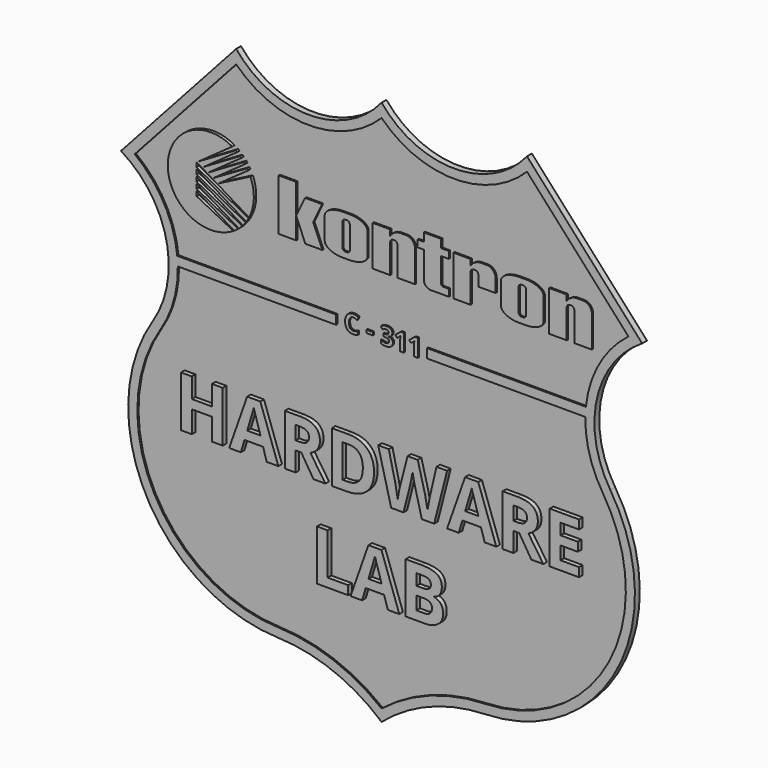
from build123d import *

# Parameters (mm, degrees)
F1_DEPTH      = 1.5
F2_DEPTH      = 0.5
F4_DEPTH      = 0.5
F5_TEXT_SIZE  = 8.0693968126
F6_DEPTH      = 0.5
F7_TEXT_SIZE  = 23.5255677177
F8_DEPTH      = 1.5
F9_DEPTH      = 1
F10_TEXT_SIZE = 23.3264580951
F11_DEPTH     = 1.5


# Not quite as in the source:
# - Text() gives the source's letters only with a copy of the font that has no kerning and outlines rounded to 1/6400 em; it was checked with that copy


with BuildPart() as f1:
    # F0 (on Front) → F1 (new body)
    with BuildSketch(Plane.XZ):
        with BuildLine():
            Line((156.4623748512, 13), (118.4623748512, 55))
            ThreePointArc((118.4623748512, 55), (94.4623748512, 43.6214168703), (70.4623748512, 55))
            ThreePointArc((70.4623748512, 55), (46.4623748512, 43.6214168703), (22.4623748512, 55))
            Line((22.4623748512, 55), (-15.5376251488, 13))
            ThreePointArc((-15.5376251488, 13), (-0.6111192408, -7.7912323471), (-5.0376251488, -33))
            ThreePointArc((-5.0376251488, -33), (-7.3094849926, -84.3223540765), (36.2328714478, -111.5842060078))
            ThreePointArc((36.2328714478, -111.5842060078), (54.4964482859, -115.3218559064), (70.4623748512, -124.9456521739))
            ThreePointArc((70.4623748512, -124.9456521739), (86.4283014165, -115.3218559064), (104.6918782546, -111.5842060078))
            ThreePointArc((104.6918782546, -111.5842060078), (148.234234695, -84.3223540765), (145.9623748512, -33))
            ThreePointArc((145.9623748512, -33), (141.5358689433, -7.7912323471), (156.4623748512, 13))
        make_face()
        with BuildLine():
            ThreePointArc((27.5723614134, 19.745571844), (28.6903368347, 13.6762247438), (27.1279654253, 7.7058111194))
            Line((27.1279654253, 7.7058111194), (9.8, 18.2))
            Line((9.8, 18.2), (9.8, 16.7))
            Line((9.8, 16.7), (26.9879537237, 7.4404873108))
            ThreePointArc((26.9879537237, 7.4404873108), (26.614342533, 6.7917137614), (26.2070574809, 6.1635327949))
            Line((26.2070574809, 6.1635327949), (9.8, 16.1))
            Line((9.8, 16.1), (9.8, 14.6))
            Line((9.8, 14.6), (26.0346697714, 5.9180078927))
            ThreePointArc((26.0346697714, 5.9180078927), (25.5780217671, 5.3164515126), (25.0900363512, 4.7400248372))
            Line((25.0900363512, 4.7400248372), (9.8, 14))
            Line((9.8, 14), (9.8, 12.5))
            Line((9.8, 12.5), (24.8878254934, 4.5184153406))
            ThreePointArc((24.8878254934, 4.5184153406), (24.3423672704, 3.9643853866), (23.7674037222, 3.4410396297))
            Line((23.7674037222, 3.4410396297), (9.8, 11.9))
            Line((9.8, 11.9), (9.8, 10.4))
            Line((9.8, 10.4), (23.5380462181, 3.2476614114))
            ThreePointArc((23.5380462181, 3.2476614114), (22.8915080931, 2.7447570116), (22.2170485866, 2.2799680742))
            Line((22.2170485866, 2.2799680742), (9.8, 9.8))
            Line((9.8, 9.8), (9.8, 8.3))
            Line((9.8, 8.3), (21.9635087632, 2.1196011265))
            ThreePointArc((21.9635087632, 2.1196011265), (0.3018885432, 13.968416191), (21.5655593046, 26.5173808788))
            Line((21.5655593046, 26.5173808788), (10.3, 18.4817355208))
            Line((10.3, 18.4817355208), (22.7054346966, 25.7892554308))
            ThreePointArc((22.7054346966, 25.7892554308), (22.9484467099, 25.6133145137), (23.1876874226, 25.4322788092))
            Line((23.1876874226, 25.4322788092), (12, 17.4521789249))
            Line((12, 17.4521789249), (24.1596372379, 24.6082375277))
            ThreePointArc((24.1596372379, 24.6082375277), (24.3773735981, 24.4018376189), (24.5907007992, 24.1908837137))
            Line((24.5907007992, 24.1908837137), (13.7, 16.422622329))
            Line((13.7, 16.422622329), (25.420447696, 23.2765534273))
            ThreePointArc((25.420447696, 23.2765534273), (25.6097684786, 23.043813903), (25.7941299736, 22.8071265901))
            Line((25.7941299736, 22.8071265901), (15.4, 15.3930657331))
            Line((15.4, 15.3930657331), (26.4951006995, 21.79983942))
            ThreePointArc((26.4951006995, 21.79983942), (26.6529834417, 21.5447255541), (26.8054412158, 21.2863330774))
            Line((26.8054412158, 21.2863330774), (17.1, 14.3635091373))
            Line((17.1, 14.3635091373), (27.5723614134, 19.745571844))
        make_face(mode=Mode.SUBTRACT)
        Polygon((42.3, 5.8), (36.5, 5.8), (36.5, 22.8), (42.3, 22.8), (42.3, 13.1), (45.2263955314, 19.1), (50.8263955314, 19.1), (47.9, 12.9), (50.9137711951, 5.8), (45.3137711951, 5.8), (42.3, 12.9), align=None, mode=Mode.SUBTRACT)
        with BuildLine():
            Line((51.7, 8.8), (51.7, 16.1))
            add(Edge.make_bspline(
                [(57.5, 19.1), (51.7, 19.1), (51.7, 16.1)],
                knots=[4.7123889804, 4.7123889804, 4.7123889804, 6.2831853072, 6.2831853072, 6.2831853072], degree=2, weights=[1, 0.7071067812, 1]))
            Line((57.5, 19.1), (60, 19.1))
            add(Edge.make_bspline(
                [(65.8, 16.1), (65.8, 19.1), (60, 19.1)],
                knots=[3.1415926536, 3.1415926536, 3.1415926536, 4.7123889804, 4.7123889804, 4.7123889804], degree=2, weights=[1, 0.7071067812, 1]))
            Line((65.8, 16.1), (65.8, 8.8))
            add(Edge.make_bspline(
                [(60, 5.8), (65.8, 5.8), (65.8, 8.8)],
                knots=[4.7123889804, 4.7123889804, 4.7123889804, 6.2831853072, 6.2831853072, 6.2831853072], degree=2, weights=[1, 0.7071067812, 1]))
            Line((60, 5.8), (57.5, 5.8))
            add(Edge.make_bspline(
                [(51.7, 8.8), (51.7, 5.8), (57.5, 5.8)],
                knots=[3.1415926536, 3.1415926536, 3.1415926536, 4.7123889804, 4.7123889804, 4.7123889804], degree=2, weights=[1, 0.7071067812, 1]))
        make_face(mode=Mode.SUBTRACT)
        with BuildLine():
            Line((67.5, 5.8), (67.5, 19.1))
            Line((67.5, 19.1), (73.3, 19.1))
            Line((73.3, 19.1), (73.3, 17.2))
            ThreePointArc((73.3, 17.2), (74.7550500371, 18.5928498393), (76.7044089061, 19.1))
            Line((76.7044089061, 19.1), (78.6002400503, 19.1))
            ThreePointArc((78.6002400503, 19.1), (80.6508497158, 18.2506096654), (81.5002400503, 16.2))
            Line((81.5002400503, 16.2), (81.5002400503, 5.8))
            Line((81.5002400503, 5.8), (75.7002400503, 5.8))
            Line((75.7002400503, 5.8), (75.7002400503, 15.4))
            ThreePointArc((75.7002400503, 15.4), (75.4073468315, 16.1071067812), (74.7002400503, 16.4))
            Line((74.7002400503, 16.4), (74.3, 16.4))
            ThreePointArc((74.3, 16.4), (73.5928932188, 16.1071067812), (73.3, 15.4))
            Line((73.3, 15.4), (73.3, 5.8))
            Line((73.3, 5.8), (67.5, 5.8))
        make_face(mode=Mode.SUBTRACT)
        with BuildLine():
            Line((84.4002400503, 16.8), (82.4002400503, 16.8))
            Line((82.4002400503, 16.8), (82.4002400503, 19.1))
            Line((82.4002400503, 19.1), (84.4002400503, 19.1))
            Line((84.4002400503, 19.1), (84.4002400503, 21.8))
            Line((84.4002400503, 21.8), (90.1002400503, 21.8))
            Line((90.1002400503, 21.8), (90.1002400503, 19.1))
            Line((90.1002400503, 19.1), (92.6768170513, 19.1))
            Line((92.6768170513, 19.1), (92.6768170513, 16.8))
            Line((92.6768170513, 16.8), (90.1002400503, 16.8))
            Line((90.1002400503, 16.8), (90.1002400503, 8.8))
            ThreePointArc((90.1002400503, 8.8), (90.3052653035, 8.3050252532), (90.8002400503, 8.1))
            Line((90.8002400503, 8.1), (92.6768170513, 8.1))
            Line((92.6768170513, 8.1), (92.6768170513, 5.8))
            Line((92.6768170513, 5.8), (86.7002400503, 5.8))
            ThreePointArc((86.7002400503, 5.8), (85.0738944536, 6.4736544033), (84.4002400503, 8.1))
            Line((84.4002400503, 8.1), (84.4002400503, 16.8))
        make_face(mode=Mode.SUBTRACT)
        with BuildLine():
            Line((94.1768170513, 5.8), (94.1768170513, 19.1))
            Line((94.1768170513, 19.1), (99.8768170513, 19.1))
            Line((99.8768170513, 19.1), (99.8768170513, 17.2))
            ThreePointArc((99.8768170513, 17.2), (101.3318670884, 18.5928498393), (103.2812259574, 19.1))
            Line((103.2812259574, 19.1), (105.1768170513, 19.1))
            ThreePointArc((105.1768170513, 19.1), (107.2274267167, 18.2506096654), (108.0768170513, 16.2))
            Line((108.0768170513, 16.2), (108.0768170513, 11.9))
            Line((108.0768170513, 11.9), (102.3768170513, 11.9))
            Line((102.3768170513, 11.9), (102.3768170513, 15.4))
            ThreePointArc((102.3768170513, 15.4), (102.0839238324, 16.1071067812), (101.3768170513, 16.4))
            Line((101.3768170513, 16.4), (100.8768170513, 16.4))
            ThreePointArc((100.8768170513, 16.4), (100.1697102701, 16.1071067812), (99.8768170513, 15.4))
            Line((99.8768170513, 15.4), (99.8768170513, 5.8))
            Line((99.8768170513, 5.8), (94.1768170513, 5.8))
        make_face(mode=Mode.SUBTRACT)
        with BuildLine():
            add(Edge.make_bspline(
                [(123.9768170513, 16.1), (123.9768170513, 19.1), (118.1768170513, 19.1)],
                knots=[0, 0, 0, 1.5707963268, 1.5707963268, 1.5707963268], degree=2, weights=[1, 0.7071067812, 1]))
            Line((123.9768170513, 16.1), (123.9768170513, 8.8))
            add(Edge.make_bspline(
                [(118.1768170513, 5.8), (123.9768170513, 5.8), (123.9768170513, 8.8)],
                knots=[4.7123889804, 4.7123889804, 4.7123889804, 6.2831853072, 6.2831853072, 6.2831853072], degree=2, weights=[1, 0.7071067812, 1]))
            Line((118.1768170513, 5.8), (115.6768170513, 5.8))
            add(Edge.make_bspline(
                [(109.8768170513, 8.8), (109.8768170513, 5.8), (115.6768170513, 5.8)],
                knots=[3.1415926536, 3.1415926536, 3.1415926536, 4.7123889804, 4.7123889804, 4.7123889804], degree=2, weights=[1, 0.7071067812, 1]))
            Line((109.8768170513, 8.8), (109.8768170513, 16.1))
            add(Edge.make_bspline(
                [(115.6768170513, 19.1), (109.8768170513, 19.1), (109.8768170513, 16.1)],
                knots=[4.7123889804, 4.7123889804, 4.7123889804, 6.2831853072, 6.2831853072, 6.2831853072], degree=2, weights=[1, 0.7071067812, 1]))
            Line((115.6768170513, 19.1), (118.1768170513, 19.1))
        make_face(mode=Mode.SUBTRACT)
        with BuildLine():
            Line((125.7768170513, 5.8), (125.7768170513, 19.1))
            Line((125.7768170513, 19.1), (131.5768170513, 19.1))
            Line((131.5768170513, 19.1), (131.5768170513, 17.2))
            ThreePointArc((131.5768170513, 17.2), (133.0318670884, 18.5928498393), (134.9812259574, 19.1))
            Line((134.9812259574, 19.1), (136.9768170513, 19.1))
            ThreePointArc((136.9768170513, 19.1), (139.0274267167, 18.2506096654), (139.8768170513, 16.2))
            Line((139.8768170513, 16.2), (139.8768170513, 5.8))
            Line((139.8768170513, 5.8), (134.0768170513, 5.8))
            Line((134.0768170513, 5.8), (134.0768170513, 15.4))
            ThreePointArc((134.0768170513, 15.4), (133.7839238324, 16.1071067812), (133.0768170513, 16.4))
            Line((133.0768170513, 16.4), (132.5768170513, 16.4))
            ThreePointArc((132.5768170513, 16.4), (131.8697102701, 16.1071067812), (131.5768170513, 15.4))
            Line((131.5768170513, 15.4), (131.5768170513, 5.8))
            Line((131.5768170513, 5.8), (125.7768170513, 5.8))
        make_face(mode=Mode.SUBTRACT)
        with BuildLine():
            Line((9.8, 18.2), (27.1279654253, 7.7058111194))
            ThreePointArc((27.1279654253, 7.7058111194), (28.6903368347, 13.6762247438), (27.5723614134, 19.745571844))
            Line((27.5723614134, 19.745571844), (17.1, 14.3635091373))
            Line((17.1, 14.3635091373), (26.8054412158, 21.2863330774))
            ThreePointArc((26.8054412158, 21.2863330774), (26.6529834417, 21.5447255541), (26.4951006995, 21.79983942))
            Line((26.4951006995, 21.79983942), (15.4, 15.3930657331))
            Line((15.4, 15.3930657331), (25.7941299736, 22.8071265901))
            ThreePointArc((25.7941299736, 22.8071265901), (25.6097684786, 23.043813903), (25.420447696, 23.2765534273))
            Line((25.420447696, 23.2765534273), (13.7, 16.422622329))
            Line((13.7, 16.422622329), (24.5907007992, 24.1908837137))
            ThreePointArc((24.5907007992, 24.1908837137), (24.3773735981, 24.4018376189), (24.1596372379, 24.6082375277))
            Line((24.1596372379, 24.6082375277), (12, 17.4521789249))
            Line((12, 17.4521789249), (23.1876874226, 25.4322788092))
            ThreePointArc((23.1876874226, 25.4322788092), (22.9484467099, 25.6133145137), (22.7054346966, 25.7892554308))
            Line((22.7054346966, 25.7892554308), (10.3, 18.4817355208))
            Line((10.3, 18.4817355208), (21.5655593046, 26.5173808788))
            ThreePointArc((21.5655593046, 26.5173808788), (0.3018885432, 13.968416191), (21.9635087632, 2.1196011265))
            Line((21.9635087632, 2.1196011265), (9.8, 8.3))
            Line((9.8, 8.3), (9.8, 9.8))
            Line((9.8, 9.8), (22.2170485866, 2.2799680742))
            ThreePointArc((22.2170485866, 2.2799680742), (22.8915080931, 2.7447570116), (23.5380462181, 3.2476614114))
            Line((23.5380462181, 3.2476614114), (9.8, 10.4))
            Line((9.8, 10.4), (9.8, 11.9))
            Line((9.8, 11.9), (23.7674037222, 3.4410396297))
            ThreePointArc((23.7674037222, 3.4410396297), (24.3423672704, 3.9643853866), (24.8878254934, 4.5184153406))
            Line((24.8878254934, 4.5184153406), (9.8, 12.5))
            Line((9.8, 12.5), (9.8, 14))
            Line((9.8, 14), (25.0900363512, 4.7400248372))
            ThreePointArc((25.0900363512, 4.7400248372), (25.5780217671, 5.3164515126), (26.0346697714, 5.9180078927))
            Line((26.0346697714, 5.9180078927), (9.8, 14.6))
            Line((9.8, 14.6), (9.8, 16.1))
            Line((9.8, 16.1), (26.2070574809, 6.1635327949))
            ThreePointArc((26.2070574809, 6.1635327949), (26.614342533, 6.7917137614), (26.9879537237, 7.4404873108))
            Line((26.9879537237, 7.4404873108), (9.8, 16.7))
            Line((9.8, 16.7), (9.8, 18.2))
        make_face()
        Polygon((36.5, 22.8), (36.5, 5.8), (42.3, 5.8), (42.3, 12.9), (45.3137711951, 5.8), (50.9137711951, 5.8), (47.9, 12.9), (50.8263955314, 19.1), (45.2263955314, 19.1), (42.3, 13.1), (42.3, 22.8), align=None)
        with BuildLine():
            add(Edge.make_bspline(
                [(57.5, 19.1), (51.7, 19.1), (51.7, 16.1)],
                knots=[4.7123889804, 4.7123889804, 4.7123889804, 6.2831853072, 6.2831853072, 6.2831853072], degree=2, weights=[1, 0.7071067812, 1]))
            Line((51.7, 16.1), (51.7, 8.8))
            add(Edge.make_bspline(
                [(51.7, 8.8), (51.7, 5.8), (57.5, 5.8)],
                knots=[3.1415926536, 3.1415926536, 3.1415926536, 4.7123889804, 4.7123889804, 4.7123889804], degree=2, weights=[1, 0.7071067812, 1]))
            Line((57.5, 5.8), (60, 5.8))
            add(Edge.make_bspline(
                [(60, 5.8), (65.8, 5.8), (65.8, 8.8)],
                knots=[4.7123889804, 4.7123889804, 4.7123889804, 6.2831853072, 6.2831853072, 6.2831853072], degree=2, weights=[1, 0.7071067812, 1]))
            Line((65.8, 8.8), (65.8, 16.1))
            add(Edge.make_bspline(
                [(65.8, 16.1), (65.8, 19.1), (60, 19.1)],
                knots=[3.1415926536, 3.1415926536, 3.1415926536, 4.7123889804, 4.7123889804, 4.7123889804], degree=2, weights=[1, 0.7071067812, 1]))
            Line((60, 19.1), (57.5, 19.1))
        make_face()
        with BuildLine():
            ThreePointArc((58.5, 7.8), (57.7928932188, 8.0928932188), (57.5, 8.8))
            Line((57.5, 8.8), (57.5, 16.1))
            ThreePointArc((57.5, 16.1), (57.7928932188, 16.8071067812), (58.5, 17.1))
            Line((58.5, 17.1), (59, 17.1))
            ThreePointArc((59, 17.1), (59.7071067812, 16.8071067812), (60, 16.1))
            Line((60, 16.1), (60, 8.8))
            ThreePointArc((60, 8.8), (59.7071067812, 8.0928932188), (59, 7.8))
            Line((59, 7.8), (58.5, 7.8))
        make_face(mode=Mode.SUBTRACT)
        with BuildLine():
            Line((73.3, 19.1), (67.5, 19.1))
            Line((67.5, 19.1), (67.5, 5.8))
            Line((67.5, 5.8), (73.3, 5.8))
            Line((73.3, 5.8), (73.3, 15.4))
            ThreePointArc((73.3, 15.4), (73.5928932188, 16.1071067812), (74.3, 16.4))
            Line((74.3, 16.4), (74.7002400503, 16.4))
            ThreePointArc((74.7002400503, 16.4), (75.4073468315, 16.1071067812), (75.7002400503, 15.4))
            Line((75.7002400503, 15.4), (75.7002400503, 5.8))
            Line((75.7002400503, 5.8), (81.5002400503, 5.8))
            Line((81.5002400503, 5.8), (81.5002400503, 16.2))
            ThreePointArc((81.5002400503, 16.2), (80.6508497158, 18.2506096654), (78.6002400503, 19.1))
            Line((78.6002400503, 19.1), (76.7044089061, 19.1))
            ThreePointArc((76.7044089061, 19.1), (74.7550500371, 18.5928498393), (73.3, 17.2))
            Line((73.3, 17.2), (73.3, 19.1))
        make_face()
        with BuildLine():
            Line((82.4002400503, 19.1), (82.4002400503, 16.8))
            Line((82.4002400503, 16.8), (84.4002400503, 16.8))
            Line((84.4002400503, 16.8), (84.4002400503, 8.1))
            ThreePointArc((84.4002400503, 8.1), (85.0738944536, 6.4736544033), (86.7002400503, 5.8))
            Line((86.7002400503, 5.8), (92.6768170513, 5.8))
            Line((92.6768170513, 5.8), (92.6768170513, 8.1))
            Line((92.6768170513, 8.1), (90.8002400503, 8.1))
            ThreePointArc((90.8002400503, 8.1), (90.3052653035, 8.3050252532), (90.1002400503, 8.8))
            Line((90.1002400503, 8.8), (90.1002400503, 16.8))
            Line((90.1002400503, 16.8), (92.6768170513, 16.8))
            Line((92.6768170513, 16.8), (92.6768170513, 19.1))
            Line((92.6768170513, 19.1), (90.1002400503, 19.1))
            Line((90.1002400503, 19.1), (90.1002400503, 21.8))
            Line((90.1002400503, 21.8), (84.4002400503, 21.8))
            Line((84.4002400503, 21.8), (84.4002400503, 19.1))
            Line((84.4002400503, 19.1), (82.4002400503, 19.1))
        make_face()
        with BuildLine():
            Line((57.5, 16.1), (57.5, 8.8))
            ThreePointArc((57.5, 8.8), (57.7928932188, 8.0928932188), (58.5, 7.8))
            Line((58.5, 7.8), (59, 7.8))
            ThreePointArc((59, 7.8), (59.7071067812, 8.0928932188), (60, 8.8))
            Line((60, 8.8), (60, 16.1))
            ThreePointArc((60, 16.1), (59.7071067812, 16.8071067812), (59, 17.1))
            Line((59, 17.1), (58.5, 17.1))
            ThreePointArc((58.5, 17.1), (57.7928932188, 16.8071067812), (57.5, 16.1))
        make_face()
        with BuildLine():
            Line((99.8768170513, 19.1), (94.1768170513, 19.1))
            Line((94.1768170513, 19.1), (94.1768170513, 5.8))
            Line((94.1768170513, 5.8), (99.8768170513, 5.8))
            Line((99.8768170513, 5.8), (99.8768170513, 15.4))
            ThreePointArc((99.8768170513, 15.4), (100.1697102701, 16.1071067812), (100.8768170513, 16.4))
            Line((100.8768170513, 16.4), (101.3768170513, 16.4))
            ThreePointArc((101.3768170513, 16.4), (102.0839238324, 16.1071067812), (102.3768170513, 15.4))
            Line((102.3768170513, 15.4), (102.3768170513, 11.9))
            Line((102.3768170513, 11.9), (108.0768170513, 11.9))
            Line((108.0768170513, 11.9), (108.0768170513, 16.2))
            ThreePointArc((108.0768170513, 16.2), (107.2274267167, 18.2506096654), (105.1768170513, 19.1))
            Line((105.1768170513, 19.1), (103.2812259574, 19.1))
            ThreePointArc((103.2812259574, 19.1), (101.3318670884, 18.5928498393), (99.8768170513, 17.2))
            Line((99.8768170513, 17.2), (99.8768170513, 19.1))
        make_face()
        with BuildLine():
            Line((123.9768170513, 8.8), (123.9768170513, 16.1))
            add(Edge.make_bspline(
                [(123.9768170513, 16.1), (123.9768170513, 19.1), (118.1768170513, 19.1)],
                knots=[0, 0, 0, 1.5707963268, 1.5707963268, 1.5707963268], degree=2, weights=[1, 0.7071067812, 1]))
            Line((118.1768170513, 19.1), (115.6768170513, 19.1))
            add(Edge.make_bspline(
                [(115.6768170513, 19.1), (109.8768170513, 19.1), (109.8768170513, 16.1)],
                knots=[4.7123889804, 4.7123889804, 4.7123889804, 6.2831853072, 6.2831853072, 6.2831853072], degree=2, weights=[1, 0.7071067812, 1]))
            Line((109.8768170513, 16.1), (109.8768170513, 8.8))
            add(Edge.make_bspline(
                [(109.8768170513, 8.8), (109.8768170513, 5.8), (115.6768170513, 5.8)],
                knots=[3.1415926536, 3.1415926536, 3.1415926536, 4.7123889804, 4.7123889804, 4.7123889804], degree=2, weights=[1, 0.7071067812, 1]))
            Line((115.6768170513, 5.8), (118.1768170513, 5.8))
            add(Edge.make_bspline(
                [(118.1768170513, 5.8), (123.9768170513, 5.8), (123.9768170513, 8.8)],
                knots=[4.7123889804, 4.7123889804, 4.7123889804, 6.2831853072, 6.2831853072, 6.2831853072], degree=2, weights=[1, 0.7071067812, 1]))
        make_face()
        with BuildLine():
            Line((115.6768170513, 8.8), (115.6768170513, 16.1))
            ThreePointArc((115.6768170513, 16.1), (115.9697102701, 16.8071067812), (116.6768170513, 17.1))
            Line((116.6768170513, 17.1), (117.1768170513, 17.1))
            ThreePointArc((117.1768170513, 17.1), (117.8839238324, 16.8071067812), (118.1768170513, 16.1))
            Line((118.1768170513, 16.1), (118.1768170513, 8.8))
            ThreePointArc((118.1768170513, 8.8), (117.8839238324, 8.0928932188), (117.1768170513, 7.8))
            Line((117.1768170513, 7.8), (116.6768170513, 7.8))
            ThreePointArc((116.6768170513, 7.8), (115.9697102701, 8.0928932188), (115.6768170513, 8.8))
        make_face(mode=Mode.SUBTRACT)
        with BuildLine():
            ThreePointArc((116.6768170513, 17.1), (115.9697102701, 16.8071067812), (115.6768170513, 16.1))
            Line((115.6768170513, 16.1), (115.6768170513, 8.8))
            ThreePointArc((115.6768170513, 8.8), (115.9697102701, 8.0928932188), (116.6768170513, 7.8))
            Line((116.6768170513, 7.8), (117.1768170513, 7.8))
            ThreePointArc((117.1768170513, 7.8), (117.8839238324, 8.0928932188), (118.1768170513, 8.8))
            Line((118.1768170513, 8.8), (118.1768170513, 16.1))
            ThreePointArc((118.1768170513, 16.1), (117.8839238324, 16.8071067812), (117.1768170513, 17.1))
            Line((117.1768170513, 17.1), (116.6768170513, 17.1))
        make_face()
        with BuildLine():
            Line((131.5768170513, 19.1), (125.7768170513, 19.1))
            Line((125.7768170513, 19.1), (125.7768170513, 5.8))
            Line((125.7768170513, 5.8), (131.5768170513, 5.8))
            Line((131.5768170513, 5.8), (131.5768170513, 15.4))
            ThreePointArc((131.5768170513, 15.4), (131.8697102701, 16.1071067812), (132.5768170513, 16.4))
            Line((132.5768170513, 16.4), (133.0768170513, 16.4))
            ThreePointArc((133.0768170513, 16.4), (133.7839238324, 16.1071067812), (134.0768170513, 15.4))
            Line((134.0768170513, 15.4), (134.0768170513, 5.8))
            Line((134.0768170513, 5.8), (139.8768170513, 5.8))
            Line((139.8768170513, 5.8), (139.8768170513, 16.2))
            ThreePointArc((139.8768170513, 16.2), (139.0274267167, 18.2506096654), (136.9768170513, 19.1))
            Line((136.9768170513, 19.1), (134.9812259574, 19.1))
            ThreePointArc((134.9812259574, 19.1), (133.0318670884, 18.5928498393), (131.5768170513, 17.2))
            Line((131.5768170513, 17.2), (131.5768170513, 19.1))
        make_face()
    extrude(amount=-F1_DEPTH)

    # F0 (on Front) → F2 (join)
    with BuildSketch(Plane.XZ):
        Polygon((36.5, 22.8), (36.5, 5.8), (42.3, 5.8), (42.3, 12.9), (45.3137711951, 5.8), (50.9137711951, 5.8), (47.9, 12.9), (50.8263955314, 19.1), (45.2263955314, 19.1), (42.3, 13.1), (42.3, 22.8), align=None)
        with BuildLine():
            add(Edge.make_bspline(
                [(57.5, 19.1), (51.7, 19.1), (51.7, 16.1)],
                knots=[4.7123889804, 4.7123889804, 4.7123889804, 6.2831853072, 6.2831853072, 6.2831853072], degree=2, weights=[1, 0.7071067812, 1]))
            Line((51.7, 16.1), (51.7, 8.8))
            add(Edge.make_bspline(
                [(51.7, 8.8), (51.7, 5.8), (57.5, 5.8)],
                knots=[3.1415926536, 3.1415926536, 3.1415926536, 4.7123889804, 4.7123889804, 4.7123889804], degree=2, weights=[1, 0.7071067812, 1]))
            Line((57.5, 5.8), (60, 5.8))
            add(Edge.make_bspline(
                [(60, 5.8), (65.8, 5.8), (65.8, 8.8)],
                knots=[4.7123889804, 4.7123889804, 4.7123889804, 6.2831853072, 6.2831853072, 6.2831853072], degree=2, weights=[1, 0.7071067812, 1]))
            Line((65.8, 8.8), (65.8, 16.1))
            add(Edge.make_bspline(
                [(65.8, 16.1), (65.8, 19.1), (60, 19.1)],
                knots=[3.1415926536, 3.1415926536, 3.1415926536, 4.7123889804, 4.7123889804, 4.7123889804], degree=2, weights=[1, 0.7071067812, 1]))
            Line((60, 19.1), (57.5, 19.1))
        make_face()
        with BuildLine():
            ThreePointArc((58.5, 7.8), (57.7928932188, 8.0928932188), (57.5, 8.8))
            Line((57.5, 8.8), (57.5, 16.1))
            ThreePointArc((57.5, 16.1), (57.7928932188, 16.8071067812), (58.5, 17.1))
            Line((58.5, 17.1), (59, 17.1))
            ThreePointArc((59, 17.1), (59.7071067812, 16.8071067812), (60, 16.1))
            Line((60, 16.1), (60, 8.8))
            ThreePointArc((60, 8.8), (59.7071067812, 8.0928932188), (59, 7.8))
            Line((59, 7.8), (58.5, 7.8))
        make_face(mode=Mode.SUBTRACT)
        with BuildLine():
            Line((73.3, 19.1), (67.5, 19.1))
            Line((67.5, 19.1), (67.5, 5.8))
            Line((67.5, 5.8), (73.3, 5.8))
            Line((73.3, 5.8), (73.3, 15.4))
            ThreePointArc((73.3, 15.4), (73.5928932188, 16.1071067812), (74.3, 16.4))
            Line((74.3, 16.4), (74.7002400503, 16.4))
            ThreePointArc((74.7002400503, 16.4), (75.4073468315, 16.1071067812), (75.7002400503, 15.4))
            Line((75.7002400503, 15.4), (75.7002400503, 5.8))
            Line((75.7002400503, 5.8), (81.5002400503, 5.8))
            Line((81.5002400503, 5.8), (81.5002400503, 16.2))
            ThreePointArc((81.5002400503, 16.2), (80.6508497158, 18.2506096654), (78.6002400503, 19.1))
            Line((78.6002400503, 19.1), (76.7044089061, 19.1))
            ThreePointArc((76.7044089061, 19.1), (74.7550500371, 18.5928498393), (73.3, 17.2))
            Line((73.3, 17.2), (73.3, 19.1))
        make_face()
        with BuildLine():
            Line((82.4002400503, 19.1), (82.4002400503, 16.8))
            Line((82.4002400503, 16.8), (84.4002400503, 16.8))
            Line((84.4002400503, 16.8), (84.4002400503, 8.1))
            ThreePointArc((84.4002400503, 8.1), (85.0738944536, 6.4736544033), (86.7002400503, 5.8))
            Line((86.7002400503, 5.8), (92.6768170513, 5.8))
            Line((92.6768170513, 5.8), (92.6768170513, 8.1))
            Line((92.6768170513, 8.1), (90.8002400503, 8.1))
            ThreePointArc((90.8002400503, 8.1), (90.3052653035, 8.3050252532), (90.1002400503, 8.8))
            Line((90.1002400503, 8.8), (90.1002400503, 16.8))
            Line((90.1002400503, 16.8), (92.6768170513, 16.8))
            Line((92.6768170513, 16.8), (92.6768170513, 19.1))
            Line((92.6768170513, 19.1), (90.1002400503, 19.1))
            Line((90.1002400503, 19.1), (90.1002400503, 21.8))
            Line((90.1002400503, 21.8), (84.4002400503, 21.8))
            Line((84.4002400503, 21.8), (84.4002400503, 19.1))
            Line((84.4002400503, 19.1), (82.4002400503, 19.1))
        make_face()
        with BuildLine():
            Line((99.8768170513, 19.1), (94.1768170513, 19.1))
            Line((94.1768170513, 19.1), (94.1768170513, 5.8))
            Line((94.1768170513, 5.8), (99.8768170513, 5.8))
            Line((99.8768170513, 5.8), (99.8768170513, 15.4))
            ThreePointArc((99.8768170513, 15.4), (100.1697102701, 16.1071067812), (100.8768170513, 16.4))
            Line((100.8768170513, 16.4), (101.3768170513, 16.4))
            ThreePointArc((101.3768170513, 16.4), (102.0839238324, 16.1071067812), (102.3768170513, 15.4))
            Line((102.3768170513, 15.4), (102.3768170513, 11.9))
            Line((102.3768170513, 11.9), (108.0768170513, 11.9))
            Line((108.0768170513, 11.9), (108.0768170513, 16.2))
            ThreePointArc((108.0768170513, 16.2), (107.2274267167, 18.2506096654), (105.1768170513, 19.1))
            Line((105.1768170513, 19.1), (103.2812259574, 19.1))
            ThreePointArc((103.2812259574, 19.1), (101.3318670884, 18.5928498393), (99.8768170513, 17.2))
            Line((99.8768170513, 17.2), (99.8768170513, 19.1))
        make_face()
        with BuildLine():
            Line((123.9768170513, 8.8), (123.9768170513, 16.1))
            add(Edge.make_bspline(
                [(123.9768170513, 16.1), (123.9768170513, 19.1), (118.1768170513, 19.1)],
                knots=[0, 0, 0, 1.5707963268, 1.5707963268, 1.5707963268], degree=2, weights=[1, 0.7071067812, 1]))
            Line((118.1768170513, 19.1), (115.6768170513, 19.1))
            add(Edge.make_bspline(
                [(115.6768170513, 19.1), (109.8768170513, 19.1), (109.8768170513, 16.1)],
                knots=[4.7123889804, 4.7123889804, 4.7123889804, 6.2831853072, 6.2831853072, 6.2831853072], degree=2, weights=[1, 0.7071067812, 1]))
            Line((109.8768170513, 16.1), (109.8768170513, 8.8))
            add(Edge.make_bspline(
                [(109.8768170513, 8.8), (109.8768170513, 5.8), (115.6768170513, 5.8)],
                knots=[3.1415926536, 3.1415926536, 3.1415926536, 4.7123889804, 4.7123889804, 4.7123889804], degree=2, weights=[1, 0.7071067812, 1]))
            Line((115.6768170513, 5.8), (118.1768170513, 5.8))
            add(Edge.make_bspline(
                [(118.1768170513, 5.8), (123.9768170513, 5.8), (123.9768170513, 8.8)],
                knots=[4.7123889804, 4.7123889804, 4.7123889804, 6.2831853072, 6.2831853072, 6.2831853072], degree=2, weights=[1, 0.7071067812, 1]))
        make_face()
        with BuildLine():
            Line((115.6768170513, 8.8), (115.6768170513, 16.1))
            ThreePointArc((115.6768170513, 16.1), (115.9697102701, 16.8071067812), (116.6768170513, 17.1))
            Line((116.6768170513, 17.1), (117.1768170513, 17.1))
            ThreePointArc((117.1768170513, 17.1), (117.8839238324, 16.8071067812), (118.1768170513, 16.1))
            Line((118.1768170513, 16.1), (118.1768170513, 8.8))
            ThreePointArc((118.1768170513, 8.8), (117.8839238324, 8.0928932188), (117.1768170513, 7.8))
            Line((117.1768170513, 7.8), (116.6768170513, 7.8))
            ThreePointArc((116.6768170513, 7.8), (115.9697102701, 8.0928932188), (115.6768170513, 8.8))
        make_face(mode=Mode.SUBTRACT)
        with BuildLine():
            Line((131.5768170513, 19.1), (125.7768170513, 19.1))
            Line((125.7768170513, 19.1), (125.7768170513, 5.8))
            Line((125.7768170513, 5.8), (131.5768170513, 5.8))
            Line((131.5768170513, 5.8), (131.5768170513, 15.4))
            ThreePointArc((131.5768170513, 15.4), (131.8697102701, 16.1071067812), (132.5768170513, 16.4))
            Line((132.5768170513, 16.4), (133.0768170513, 16.4))
            ThreePointArc((133.0768170513, 16.4), (133.7839238324, 16.1071067812), (134.0768170513, 15.4))
            Line((134.0768170513, 15.4), (134.0768170513, 5.8))
            Line((134.0768170513, 5.8), (139.8768170513, 5.8))
            Line((139.8768170513, 5.8), (139.8768170513, 16.2))
            ThreePointArc((139.8768170513, 16.2), (139.0274267167, 18.2506096654), (136.9768170513, 19.1))
            Line((136.9768170513, 19.1), (134.9812259574, 19.1))
            ThreePointArc((134.9812259574, 19.1), (133.0318670884, 18.5928498393), (131.5768170513, 17.2))
            Line((131.5768170513, 17.2), (131.5768170513, 19.1))
        make_face()
    extrude(amount=F2_DEPTH)

    # F3 (on face) → F4 (join)
    with BuildSketch(Plane.XZ):
        with BuildLine():
            ThreePointArc((70.4623748512, 55), (46.4623748512, 43.6214168703), (22.4623748512, 55))
            Line((22.4623748512, 55), (-15.5376251488, 13))
            ThreePointArc((-15.5376251488, 13), (-0.6111192408, -7.7912323471), (-5.0376251488, -33))
            ThreePointArc((-5.0376251488, -33), (-7.3094849926, -84.3223540765), (36.2328714478, -111.5842060078))
            ThreePointArc((36.2328714478, -111.5842060078), (54.4964482859, -115.3218559064), (70.4623748512, -124.9456521739))
            ThreePointArc((70.4623748512, -124.9456521739), (86.4283014165, -115.3218559064), (104.6918782546, -111.5842060078))
            ThreePointArc((104.6918782546, -111.5842060078), (148.234234695, -84.3223540765), (145.9623748512, -33))
            ThreePointArc((145.9623748512, -33), (141.5358689433, -7.7912323471), (156.4623748512, 13))
            Line((156.4623748512, 13), (118.4623748512, 55))
            ThreePointArc((118.4623748512, 55), (94.4623748512, 43.6214168703), (70.4623748512, 55))
        make_face()
        with BuildLine():
            Line((55.4623748512, -11.4617722872), (3.028498128, -11.4617722872))
            ThreePointArc((3.028498128, -11.4617722872), (-1.3950849575, 2.4934292598), (-11.0092982959, 13.5334763347))
            Line((-11.0092982959, 13.5334763347), (22.4670113835, 50.5336080856))
            ThreePointArc((22.4670113835, 50.5336080856), (46.4656474032, 40.6214170278), (70.4623748512, 50.5382277128))
            ThreePointArc((70.4623748512, 50.5382277128), (94.4591022992, 40.6214170278), (118.457738319, 50.5336080856))
            Line((118.457738319, 50.5336080856), (151.9340479984, 13.5334763347))
            ThreePointArc((151.9340479984, 13.5334763347), (142.3198346599, 2.4934292598), (137.8962515745, -11.4617722872))
            Line((137.8962515745, -11.4617722872), (85.4623748512, -11.4617722872))
            Line((85.4623748512, -11.4617722872), (85.4623748512, -14.4617722872))
            Line((85.4623748512, -14.4617722872), (137.7146632791, -14.4617722872))
            ThreePointArc((137.7146632791, -14.4617722872), (139.0775292529, -24.9688233143), (143.4400117804, -34.6240949908))
            ThreePointArc((143.4400117804, -34.6240949908), (145.5782328099, -82.9274870628), (104.5971914542, -108.5857006452))
            ThreePointArc((104.5971914542, -108.5857006452), (86.5280302377, -112.0774591835), (70.4623748512, -121.0541891984))
            ThreePointArc((70.4623748512, -121.0541891984), (54.3967194648, -112.0774591835), (36.3275582483, -108.5857006452))
            ThreePointArc((36.3275582483, -108.5857006452), (-4.6534831074, -82.9274870628), (-2.515262078, -34.6240949908))
            ThreePointArc((-2.515262078, -34.6240949908), (1.8472204496, -24.9688233143), (3.2100864233, -14.4617722872))
            Line((3.2100864233, -14.4617722872), (55.4623748512, -14.4617722872))
            Line((55.4623748512, -14.4617722872), (55.4623748512, -11.4617722872))
        make_face(mode=Mode.SUBTRACT)
    extrude(amount=F4_DEPTH)

    # F5 (on face) → F6 (join)
    with BuildSketch(Plane.XZ):
        with Locations((57.9623748512, -15.2717379923)):
            Text('C - 311', F5_TEXT_SIZE, font='Open Sans', font_style=FontStyle.BOLD, text_align=(TextAlign.LEFT, TextAlign.BOTTOM))
    extrude(amount=F6_DEPTH)

    # F7 (on face) → F8 (join)
    with BuildSketch(Plane.XZ):
        with Locations((2.9623748512, -61.0541891984)):
            Text('HARDWARE', F7_TEXT_SIZE, font='Open Sans', font_style=FontStyle.BOLD, text_align=(TextAlign.LEFT, TextAlign.BOTTOM))
    extrude(amount=F8_DEPTH)

    # F0 (on Front) → F9 (join)
    with BuildSketch(Plane.XZ):
        with BuildLine():
            Line((9.8, 18.2), (27.1279654253, 7.7058111194))
            ThreePointArc((27.1279654253, 7.7058111194), (28.6903368347, 13.6762247438), (27.5723614134, 19.745571844))
            Line((27.5723614134, 19.745571844), (17.1, 14.3635091373))
            Line((17.1, 14.3635091373), (26.8054412158, 21.2863330774))
            ThreePointArc((26.8054412158, 21.2863330774), (26.6529834417, 21.5447255541), (26.4951006995, 21.79983942))
            Line((26.4951006995, 21.79983942), (15.4, 15.3930657331))
            Line((15.4, 15.3930657331), (25.7941299736, 22.8071265901))
            ThreePointArc((25.7941299736, 22.8071265901), (25.6097684786, 23.043813903), (25.420447696, 23.2765534273))
            Line((25.420447696, 23.2765534273), (13.7, 16.422622329))
            Line((13.7, 16.422622329), (24.5907007992, 24.1908837137))
            ThreePointArc((24.5907007992, 24.1908837137), (24.3773735981, 24.4018376189), (24.1596372379, 24.6082375277))
            Line((24.1596372379, 24.6082375277), (12, 17.4521789249))
            Line((12, 17.4521789249), (23.1876874226, 25.4322788092))
            ThreePointArc((23.1876874226, 25.4322788092), (22.9484467099, 25.6133145137), (22.7054346966, 25.7892554308))
            Line((22.7054346966, 25.7892554308), (10.3, 18.4817355208))
            Line((10.3, 18.4817355208), (21.5655593046, 26.5173808788))
            ThreePointArc((21.5655593046, 26.5173808788), (0.3018885432, 13.968416191), (21.9635087632, 2.1196011265))
            Line((21.9635087632, 2.1196011265), (9.8, 8.3))
            Line((9.8, 8.3), (9.8, 9.8))
            Line((9.8, 9.8), (22.2170485866, 2.2799680742))
            ThreePointArc((22.2170485866, 2.2799680742), (22.8915080931, 2.7447570116), (23.5380462181, 3.2476614114))
            Line((23.5380462181, 3.2476614114), (9.8, 10.4))
            Line((9.8, 10.4), (9.8, 11.9))
            Line((9.8, 11.9), (23.7674037222, 3.4410396297))
            ThreePointArc((23.7674037222, 3.4410396297), (24.3423672704, 3.9643853866), (24.8878254934, 4.5184153406))
            Line((24.8878254934, 4.5184153406), (9.8, 12.5))
            Line((9.8, 12.5), (9.8, 14))
            Line((9.8, 14), (25.0900363512, 4.7400248372))
            ThreePointArc((25.0900363512, 4.7400248372), (25.5780217671, 5.3164515126), (26.0346697714, 5.9180078927))
            Line((26.0346697714, 5.9180078927), (9.8, 14.6))
            Line((9.8, 14.6), (9.8, 16.1))
            Line((9.8, 16.1), (26.2070574809, 6.1635327949))
            ThreePointArc((26.2070574809, 6.1635327949), (26.614342533, 6.7917137614), (26.9879537237, 7.4404873108))
            Line((26.9879537237, 7.4404873108), (9.8, 16.7))
            Line((9.8, 16.7), (9.8, 18.2))
        make_face()
    extrude(amount=F9_DEPTH)

    # F10 (on face) → F11 (join, through all)
    with BuildSketch(Plane.XZ):
        with Locations((47.8466447762, -91.0541891984)):
            Text('LAB', F10_TEXT_SIZE, font='Open Sans', font_style=FontStyle.BOLD, text_align=(TextAlign.LEFT, TextAlign.BOTTOM))
    extrude(amount=F11_DEPTH)


solid = f1.part
